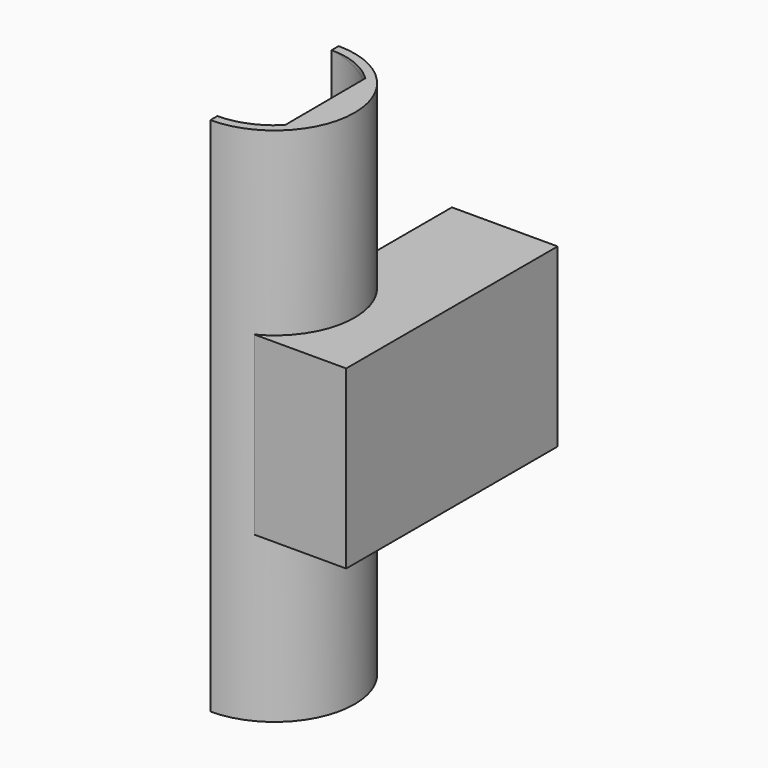
from build123d import *

# Parameters (mm, degrees)
F1_DEPTH     = 37.95141
F3_DEPTH     = 0.75946
F4_T4_DEPTH  = 76.9415838332
F4_S5_R      = 10.287
F4_T6_DEPTH  = 40
F5_W         = 23.114
F5_H         = 1.59512
F6_DEPTH     = 25.4
F9_DEPTH     = 25.4
F10_T4_DEPTH = 21.5531370707
F10_S5_R     = 10.287
F10_T6_DEPTH = 12
F14_W        = 15.24
F14_H        = 25.4
F14_W_2      = 12.7
F14_H_2      = 20.32
F15_DEPTH    = 38.1
F12_W        = 6.096
F12_H        = 20.32
F17_DEPTH    = 25.4


# Not quite as in the source:
# - a fillet or chamfer that OpenCascade refuses, or shapes differently, is made with other operations: its cross-section is extruded or revolved along the edge and cut away or added


with BuildPart() as f1:
    # F0 (on Top) → F1 (new body, symmetric)
    with BuildSketch(Plane.XY):
        with BuildLine():
            ThreePointArc((0, 10.287), (10.287, 0), (0, -10.287))
            Line((0, -10.287), (0, -11.557))
            ThreePointArc((0, -11.557), (11.557, 0), (0, 11.557))
            Line((0, 11.557), (0, 10.287))
        make_face()
    extrude(amount=F1_DEPTH, both=True)

    # F2 (on face) → F3 (join, symmetric)
    with BuildSketch(Plane.XY.offset(37.95141)):
        with BuildLine():
            Line((0, 11.557), (0, -11.557))
            ThreePointArc((0, -11.557), (11.557, 0), (0, 11.557))
        make_face()
    extrude(amount=F3_DEPTH, both=True)

    # F4: chamfer of 1.524 x 10.8438234569 on 1 edges, made by hand


with BuildPart() as f4_tool2:
    # F4_s3 → F4_t4 (new body)
    with BuildSketch(Plane.XZ.offset(-38.4707919166)):
        Polygon((0, 38.71595), (10.8438234569, 37.19195), (0, 37.19195), align=None)
    extrude(amount=F4_T4_DEPTH)

    # F4_s5 → F4_t6 (intersect, symmetric)
    with BuildSketch(Plane.XY.offset(38)):
        Circle(F4_S5_R)
    extrude(amount=F4_T6_DEPTH, both=True, mode=Mode.INTERSECT)


with BuildPart() as f1_1:
    add(f1.part)

    # F4_t1: cut F4_tool2
    add(f4_tool2.part, mode=Mode.SUBTRACT)

    # F5 (on face) → F6 (cut)
    with BuildSketch(Plane(origin=(0, 0, 0), x_dir=(0, -1, 0), z_dir=(-1, 0, 0))):
        with Locations((0, -37.15385)):
            Rectangle(F5_W, F5_H)
    extrude(amount=-F6_DEPTH, mode=Mode.SUBTRACT)

    # F8 (on face) → F9 (cut)
    with BuildSketch(Plane.XY.offset(38.71087)):
        with BuildLine():
            Line((7.0719993682, -7.4705551291), (6.9994361845, 7.5385848871))
            ThreePointArc((6.9994361845, 7.5385848871), (3.7766669941, 9.5686548384), (0.0361460782, 10.2869364954))
            Line((0.0361460782, 10.2869364954), (0.0361460782, -10.2869364954))
            ThreePointArc((0.0361460782, -10.2869364954), (3.8228829333, -9.5502845548), (7.0719993682, -7.4705551291))
        make_face()
    extrude(amount=-F9_DEPTH, mode=Mode.SUBTRACT)

    # F10: chamfer of 1.27 on 1 edges, made by hand


with BuildPart() as f10_tool2:
    # F10_s3 → F10_t4 (new body)
    with BuildSketch(Plane(origin=(0.0519758467, -10.7508066832, -0.0073047289), x_dir=(-0.9999883135, -0.0048345432, 0), z_dir=(-0.0048345421, 0.9999880827, 0.0006794506))):
        with BuildLine():
            Line((-7.0024721698, 39.0354748619), (-8.3267685678, 37.5120486506))
            Line((-8.3267685678, 37.5120486506), (-8.3232336123, 37.4868958359))
            ThreePointArc((-8.3232336123, 37.4868958359), (-7.6800684701, 37.6109410786), (-7.0322650445, 37.7019828278))
            Line((-7.0322650445, 37.7019828278), (-7.0104, 37.7271356426))
            ThreePointArc((-7.0104, 37.7271356426), (-7.0104, 38.3813052522), (-6.9770721698, 39.0354748619))
            Line((-6.9770721698, 39.0354748619), (-7.0024721698, 39.0354748619))
        make_face()
    extrude(amount=F10_T4_DEPTH)

    # F10_s5 → F10_t6 (intersect, symmetric)
    with BuildSketch(Plane.XY.offset(38.3)):
        Circle(F10_S5_R)
    extrude(amount=F10_T6_DEPTH, both=True, mode=Mode.INTERSECT)


with BuildPart() as f1_2:
    add(f1_1.part)

    # F10_t1: cut F10_tool2
    add(f10_tool2.part, mode=Mode.SUBTRACT)

    # F14 (on offset) → F15 (join)
    with BuildSketch(Plane.XZ.offset(-27.8384)):
        with Locations((10.922, 0)):
            Rectangle(F14_W, F14_H)
        with Locations((10.922, 0)):
            Rectangle(F14_W_2, F14_H_2, mode=Mode.SUBTRACT)
        with Locations((10.922, 0)):
            Rectangle(F14_W_2, F14_H_2)
    extrude(amount=F15_DEPTH)

    # F14 (on offset) → F16 section 0
    with BuildSketch(Plane.XZ.offset(-27.8384)):
        with Locations((10.922, 0)):
            Rectangle(F14_W_2, F14_H_2)
    # F12 (on offset) → F16 section 1
    with BuildSketch(Plane.XZ.offset(-10.16)):
        with Locations((7.62, 0)):
            Rectangle(F12_W, F12_H)
    loft(mode=Mode.SUBTRACT)

    # F17 (cut): a face of the model
    f17_faces = [f1_2.faces().sort_by_distance(p)[0] for p in [
        (6.1976073011, 0, -12.7),
    ]]
    extrude(f17_faces, amount=-F17_DEPTH, mode=Mode.SUBTRACT)


solid = f1_2.part
